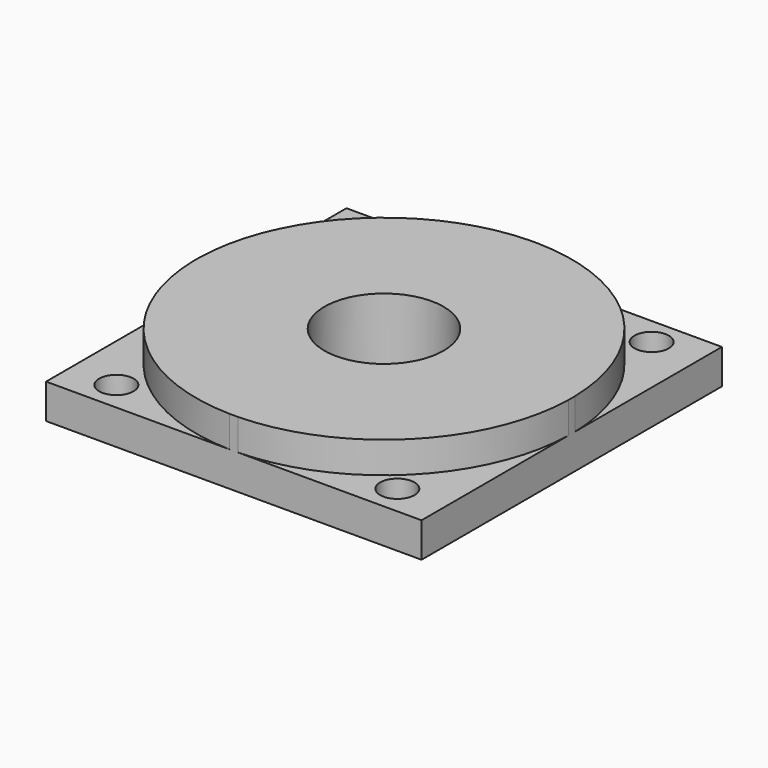
from build123d import *

# Parameters (mm, degrees)
F0_R     = 3.5
F0_R_2   = 19.05
F1_DEPTH = 11.1125
F2_R     = 5.5
F2_R_2   = 5.4991
F3_DEPTH = 9
F4_R     = 19.05
F5_DEPTH = 10


# Not quite as in the source:
# - a length typed as a fraction of an inch, garbled in the dataset ("3 / 203.2 mm" for 3/8 in), is restored


with BuildPart() as f1:
    # F0 (on Top) → F1 (new body)
    with BuildSketch(Plane.XY):
        Polygon((0, 60), (-60, 60), (-60, -60), (60, -60), (60, 0), (60, 60), align=None)
        with Locations((-45.1685115695, -50.4610737026)):
            Circle(F0_R, mode=Mode.SUBTRACT)
        with Locations((44.6352420051, -50.4610737026)):
            Circle(F0_R, mode=Mode.SUBTRACT)
        with Locations((-45.1685115695, 51.1389262974)):
            Circle(F0_R, mode=Mode.SUBTRACT)
        Circle(F0_R_2, mode=Mode.SUBTRACT)
        with Locations((44.6352420051, 51.1389262974)):
            Circle(F0_R, mode=Mode.SUBTRACT)
    extrude(amount=F1_DEPTH)

    # F2 (on face) → F3 (cut)
    with BuildSketch(Plane.XY.offset(11.1125)):
        with Locations((-45.1685115695, -50.4610737026)):
            Circle(F2_R)
        with Locations((44.6352420051, -50.4610737026)):
            Circle(F2_R_2)
        with Locations((44.6352420051, 51.1389262974)):
            Circle(F2_R_2)
        with Locations((-45.1685115695, 51.1389262974)):
            Circle(F2_R_2)
    extrude(amount=-F3_DEPTH, mode=Mode.SUBTRACT)

    # F4 (on face) → F5 (join)
    with BuildSketch(Plane.XY.offset(11.1125)):
        with BuildLine():
            Line((60, -1.3768154949), (60, 1.3768154949))
            ThreePointArc((60, 1.3768154949), (42.4375754545, 42.4375754545), (1.3768154949, 60))
            Line((1.3768154949, 60), (-1.3768154949, 60))
            ThreePointArc((-1.3768154949, 60), (-42.4375754545, 42.4375754545), (-60, 1.3768154949))
            Line((-60, 1.3768154949), (-60, -1.3768154949))
            ThreePointArc((-60, -1.3768154949), (-42.4375754545, -42.4375754545), (-1.3768154949, -60))
            Line((-1.3768154949, -60), (1.3768154949, -60))
            ThreePointArc((1.3768154949, -60), (42.4375754545, -42.4375754545), (60, -1.3768154949))
        make_face()
        Circle(F4_R, mode=Mode.SUBTRACT)
    extrude(amount=F5_DEPTH)


solid = f1.part
